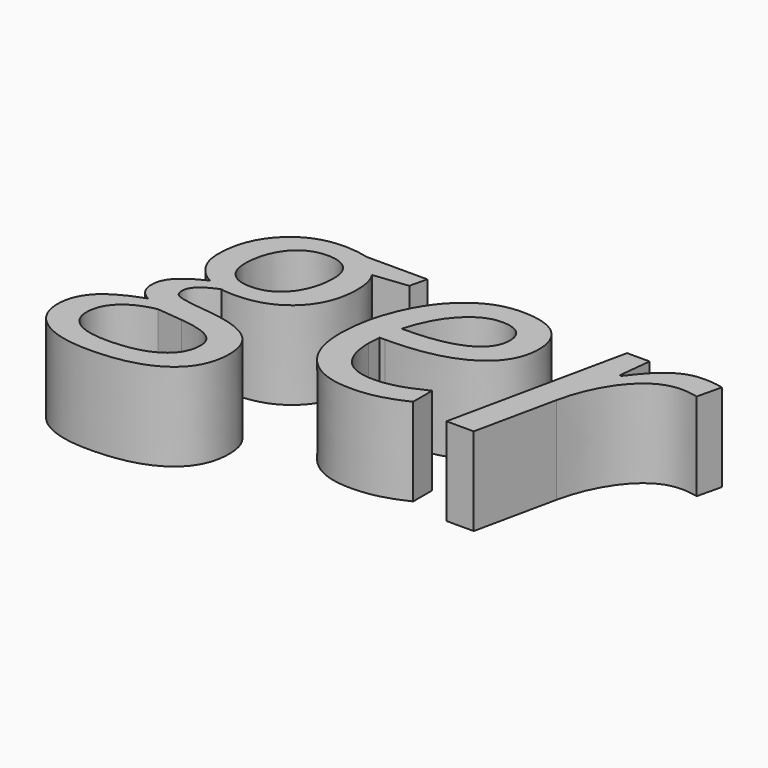
from build123d import *

# Parameters (mm, degrees)
F0_TEXT_SIZE = 37.9219871118
F1_DEPTH     = 10


# Not quite as in the source:
# - Text() gives the source's letters only with a copy of the font that has no kerning and outlines rounded to 1/6400 em; it was checked with that copy


with BuildPart() as f1:
    # F0 (on Top) → F1 (new body)
    with BuildSketch(Plane.XY):
        with Locations((6.179288961, 15.3763694689)):
            Text('ger', F0_TEXT_SIZE, font='Open Sans', font_style=FontStyle.ITALIC, text_align=(TextAlign.LEFT, TextAlign.BOTTOM))
    extrude(amount=F1_DEPTH)


solid = f1.part
